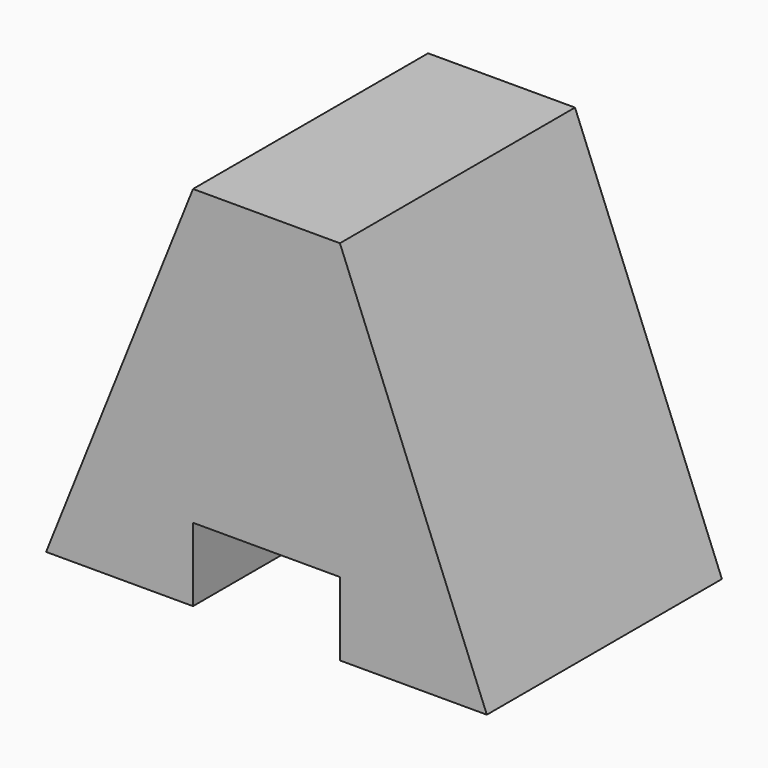
from build123d import *

# Parameters (mm, degrees)
F0_W     = 38.1
F0_H     = 31.75
F1_DEPTH = 25.4
F3_DEPTH = 25.4
F4_DEPTH = 25.4
F5_W     = 12.7
F5_H     = 6.35
F6_DEPTH = 25.401


# Not quite as in the source:
# - a feature names something its author has since deleted; it is built from what else it names


with BuildPart() as f1:
    # F0 (on Front) → F1 (new body)
    with BuildSketch(Plane.XZ):
        with Locations((19.05, 15.875)):
            Rectangle(F0_W, F0_H)
    extrude(amount=F1_DEPTH)

    # F0 (on Front) → F3 (join)
    with BuildSketch(Plane.XZ):
        with Locations((19.05, 15.875)):
            Rectangle(F0_W, F0_H)
    extrude(amount=F3_DEPTH)

    # F0 (on Front) → F4 (join)
    with BuildSketch(Plane.XZ):
        with Locations((19.05, 15.875)):
            Rectangle(F0_W, F0_H)
    extrude(amount=F4_DEPTH)

    # F5 (on face) → F6 (cut, through all)
    with BuildSketch(Plane.XZ.offset(25.4)):
        Polygon((0, 31.75), (0, 0), (12.7, 31.75), align=None)
        Polygon((38.1, 31.75), (25.4, 31.75), (38.1, 0), align=None)
        with Locations((19.05, 3.175)):
            Rectangle(F5_W, F5_H)
    extrude(amount=-F6_DEPTH, mode=Mode.SUBTRACT)


solid = f1.part
